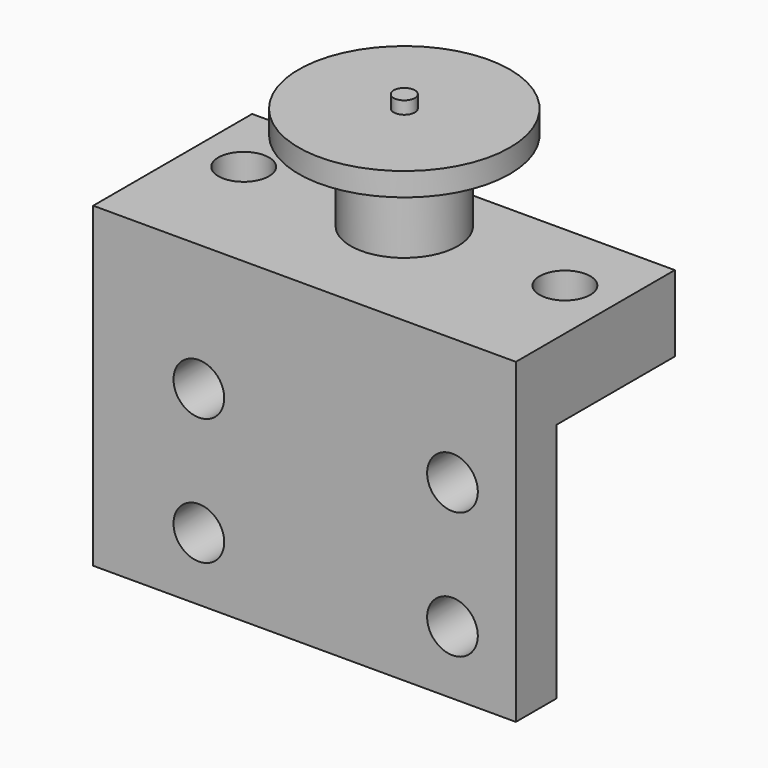
from build123d import *

# Parameters (mm, degrees)
F0_W      = 100
F0_H      = 35
F1_DEPTH  = 18
F3_D      = 12
F4_R      = 12.7
F5_DEPTH  = 19
F6_R      = 25
F6_R_2    = 12.7
F7_DEPTH  = 5.5
F8_R      = 2.5
F9_DEPTH  = 3
F10_W     = 100
F10_H     = 57
F10_H_2   = 18
F11_DEPTH = 12
F13_D     = 12


# Not quite as in the source:
# - a feature names something its author has since deleted; it is built from what else it names


with BuildPart() as f1:
    # F0 (on Top) → F1 (new body)
    with BuildSketch(Plane.XY):
        Rectangle(F0_W, F0_H)
    extrude(amount=-F1_DEPTH)

    # F3 (through all)
    with Locations(Plane.XY):
        with Locations((-38, 0), (38, 0)):
            Hole(F3_D / 2)

    # F4 (on face) → F5 (join)
    with BuildSketch(Plane.XY):
        Circle(F4_R)
    extrude(amount=F5_DEPTH)

    # F6 (on face) → F7 (join)
    with BuildSketch(Plane.XY.offset(19)):
        Circle(F6_R)
        Circle(F6_R_2, mode=Mode.SUBTRACT)
        Circle(F6_R_2)
    extrude(amount=F7_DEPTH)

    # F8 (on face) → F9 (join)
    with BuildSketch(Plane.XY.offset(24.5)):
        Circle(F8_R)
    extrude(amount=F9_DEPTH)

    # F10 (on face) → F11 (join)
    with BuildSketch(Plane.XZ.offset(17.5)):
        with Locations((0, -46.5)):
            Rectangle(F10_W, F10_H)
        with Locations((0, -9)):
            Rectangle(F10_W, F10_H_2)
    extrude(amount=F11_DEPTH)

    # F13 (through all)
    with Locations(Plane(origin=(0, -17.5, 0), x_dir=(-1, 0, 0), z_dir=(0, 1, 0))):
        with Locations((-35, -30), (-35, -60), (25, -30), (25, -60)):
            Hole(F13_D / 2)


solid = f1.part
